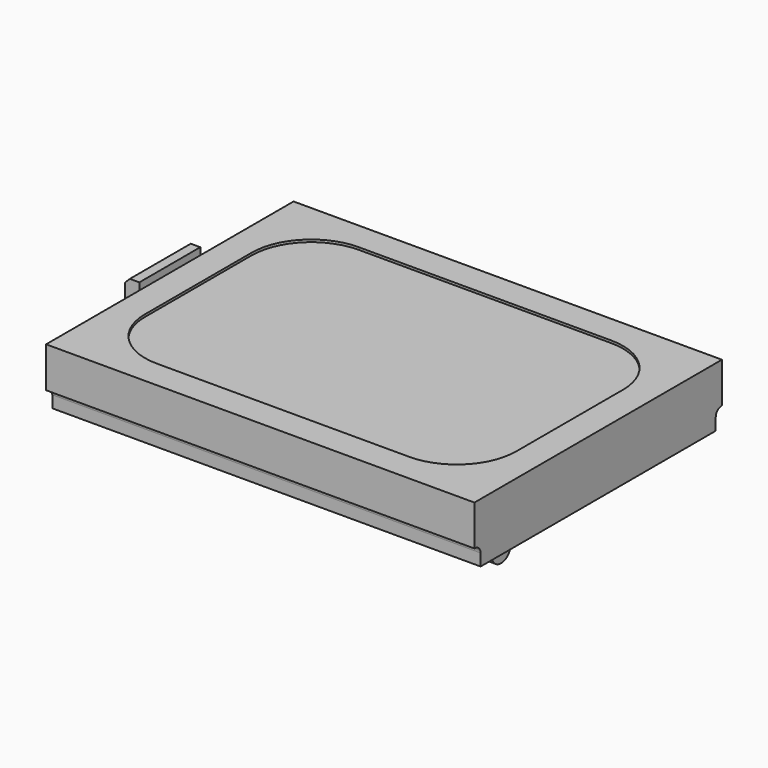
from build123d import *

# Parameters (mm, degrees)
F0_W          = 18
F0_H          = 13
F1_DEPTH      = 2.5
F3_DEPTH      = 0.1
F5_R          = 0.5
F6_DEPTH      = 0.5
F8_DEPTH      = 9.001
F8_DEPTH_BACK = 9.001
F10_DEPTH     = 1.6


# Not quite as in the source:
# - a pattern or mirror of a feature is missing from the dataset's text; its kind, count and spacing are read off the source's solid


with BuildPart() as f1:
    # F0 (on Top) → F1 (new body)
    with BuildSketch(Plane.XY):
        Rectangle(F0_W, F0_H)
    extrude(amount=F1_DEPTH)

    # F2 (on face) → F3 (cut)
    with BuildSketch(Plane.XY.offset(2.5)):
        with BuildLine():
            ThreePointArc((7.8, 2.8), (7.067766953, 4.567766953), (5.3, 5.3))
            Line((5.3, 5.3), (-5.3, 5.3))
            ThreePointArc((-5.3, 5.3), (-7.067766953, 4.567766953), (-7.8, 2.8))
            Line((-7.8, 2.8), (-7.8, -2.8))
            ThreePointArc((-7.8, -2.8), (-7.067766953, -4.567766953), (-5.3, -5.3))
            Line((-5.3, -5.3), (5.3, -5.3))
            ThreePointArc((5.3, -5.3), (7.067766953, -4.567766953), (7.8, -2.8))
            Line((7.8, -2.8), (7.8, 2.8))
        make_face()
    extrude(amount=-F3_DEPTH, mode=Mode.SUBTRACT)

    # F5 (on offset) → F6 (join, symmetric)
    with BuildSketch(Plane.YZ.offset(8.1)):
        with Locations((-4.6, -0.15)):
            Circle(F5_R)
    f6 = extrude(amount=F6_DEPTH, both=True)

    # F6_copies: F6 across plane
    add(f6.mirror(Plane(origin=(0, 0, 0), x_dir=(0, 0, -1), z_dir=(-1, 0, 0))))

    # F7 (on Right) → F8 (cut, two sides)
    with BuildSketch(Plane.YZ) as f8_sk:
        with BuildLine():
            Line((-6.5, 0.8), (-6.5, 0))
            Line((-6.5, 0), (-6.175, 0))
            Line((-6.175, 0), (-6.175, 0.5))
            ThreePointArc((-6.175, 0.5), (-6.2628679656, 0.7121320344), (-6.475, 0.8))
            Line((-6.475, 0.8), (-6.5, 0.8))
        make_face()
    f8 = extrude(amount=-F8_DEPTH, mode=Mode.SUBTRACT) + extrude(f8_sk.sketch, amount=F8_DEPTH_BACK, mode=Mode.SUBTRACT)

    # F8_copies: F8 across plane
    add(f8.mirror(Plane.ZX), mode=Mode.SUBTRACT)

    # F9 (on Front) → F10 (join, symmetric)
    with BuildSketch(Plane.XZ):
        Polygon((-9, 1.85), (-9, 2.8), (-9.4, 2.8), (-9.6, 2.6), (-9.6, 1.85), align=None)
    extrude(amount=F10_DEPTH, both=True)


solid = f1.part
